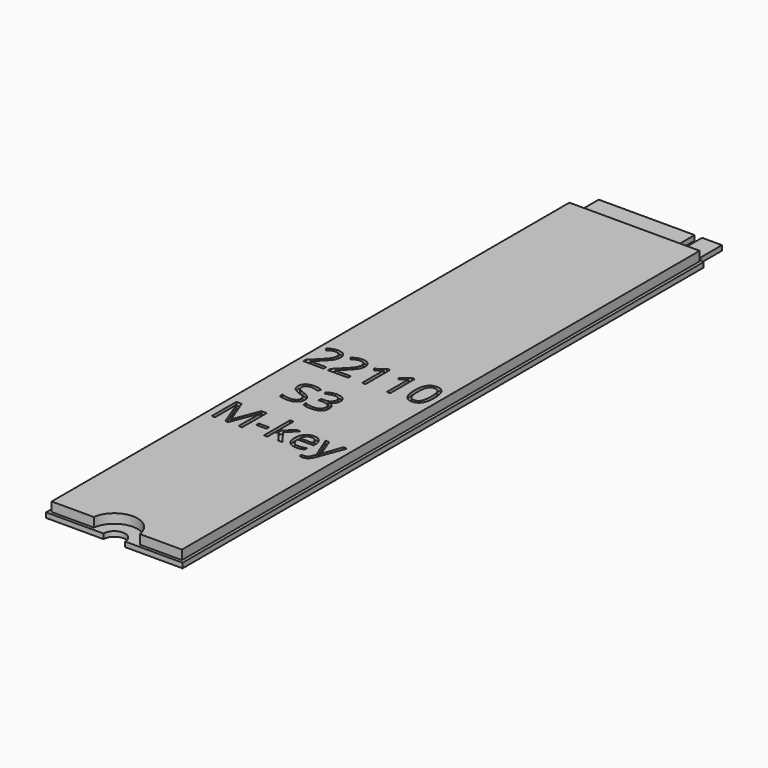
from build123d import *

# Parameters (mm, degrees)
F2_W          = 22
F2_H          = 110
F3_DEPTH      = 0.8
F4_W          = 21
F4_H          = 104.3
F5_DEPTH      = 1.5
F7_DEPTH      = 0.801
F8_R          = 1.75
F9_DEPTH      = 2.301
F11_DEPTH     = 1.5
F12_TEXT_SIZE = 6.9444444444
F13_DEPTH     = 0.5


# Not quite as in the source:
# - Text() gives the source's letters only with a copy of the font that has no kerning and outlines rounded to 1/6400 em; it was checked with that copy


with BuildPart() as f3:
    # F2 (on Top) → F3 (new body)
    with BuildSketch(Plane.XY):
        Rectangle(F2_W, F2_H)
    extrude(amount=F3_DEPTH)

    # F4 (on face) → F5 (join)
    with BuildSketch(Plane.XY.offset(0.8)):
        with Locations((0, -2.35)):
            Rectangle(F4_W, F4_H)
    extrude(amount=F5_DEPTH)

    # F6 (on face) → F7 (cut, through all)
    with BuildSketch(Plane.XY.offset(0.8)):
        with BuildLine():
            Line((-9.925, 51), (-9.925, 55))
            Line((-9.925, 55), (-11, 55))
            Line((-11, 55), (-11, 49.925))
            ThreePointArc((-11, 49.925), (-10.2398602102, 50.2398602102), (-9.925, 51))
        make_face()
        with BuildLine():
            Line((11, 55), (9.925, 55))
            Line((9.925, 55), (9.925, 51))
            ThreePointArc((9.925, 51), (10.2398602102, 50.2398602102), (11, 49.925))
            Line((11, 49.925), (11, 55))
        make_face()
        with BuildLine():
            Line((5.53, 55), (5.53, 51.6))
            ThreePointArc((5.53, 51.6), (6.13, 51), (6.73, 51.6))
            Line((6.73, 51.6), (6.73, 55))
            Line((6.73, 55), (5.53, 55))
        make_face()
    extrude(amount=-F7_DEPTH, mode=Mode.SUBTRACT)

    # F8 (on face) → F9 (cut, through all)
    with BuildSketch(Plane(origin=(0, 0, 0), x_dir=(1, 0, 0), z_dir=(0, 0, -1))):
        with Locations((0, 55)):
            Circle(F8_R)
    extrude(amount=-F9_DEPTH, mode=Mode.SUBTRACT)

    # F10 (on face) → F11 (cut, through all)
    with BuildSketch(Plane.XY.offset(2.3)):
        with BuildLine():
            ThreePointArc((-1.6770509831, -54.5), (0, -53.25), (1.6770509831, -54.5))
            Line((1.6770509831, -54.5), (3.7165171868, -54.5))
            ThreePointArc((3.7165171868, -54.5), (0, -51.25), (-3.7165171868, -54.5))
            Line((-3.7165171868, -54.5), (-1.6770509831, -54.5))
        make_face()
    extrude(amount=-F11_DEPTH, mode=Mode.SUBTRACT)

    # F12 (on face) → F13 (cut)
    with BuildSketch(Plane.XY.offset(2.3)):
        with Locations((-9.9940321181, -4.85)):
            Text('22110', F12_TEXT_SIZE, font='Open Sans', text_align=(TextAlign.LEFT, TextAlign.BOTTOM))
        with Locations((-6.3850911458, -14.2944444444)):
            Text('S3', F12_TEXT_SIZE, font='Open Sans', text_align=(TextAlign.LEFT, TextAlign.BOTTOM))
        with Locations((-9.9940321181, -23.7388888889)):
            Text('M-key', F12_TEXT_SIZE, font='Open Sans', text_align=(TextAlign.LEFT, TextAlign.BOTTOM))
    extrude(amount=-F13_DEPTH, mode=Mode.SUBTRACT)


solid = f3.part
